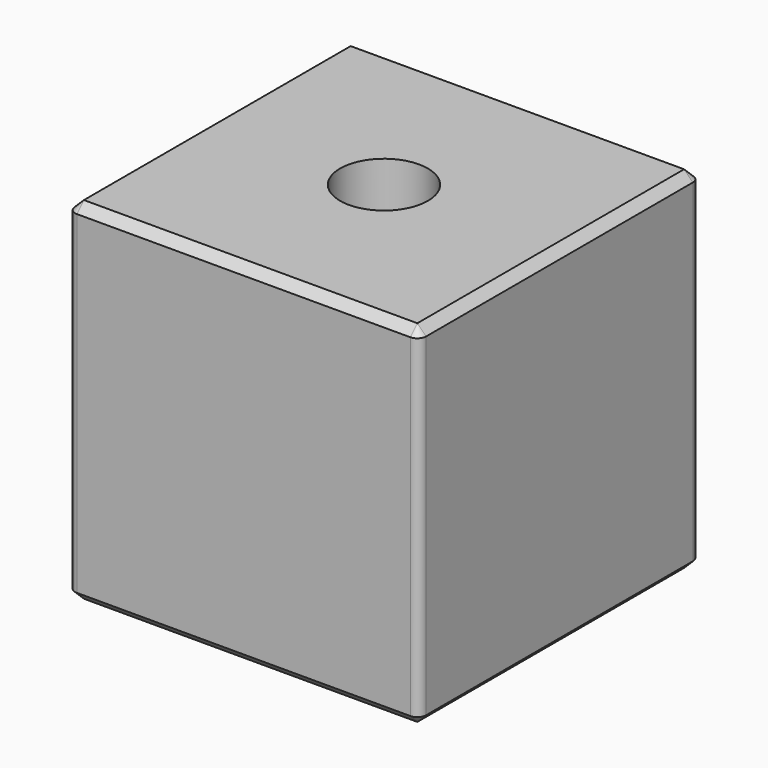
from build123d import *

# Parameters (mm, degrees)
F0_R     = 12.5
F1_DEPTH = 50
F2_SIZE  = 2.49999


# Not quite as in the source:
# - a fillet or chamfer is up to 0.001 mm smaller than in the source, because OpenCascade refuses the exact size


with BuildPart() as f1:
    # F0 (on Top) → F1 (new body, symmetric)
    with BuildSketch(Plane.XY):
        with BuildLine():
            ThreePointArc((-50, -47.5), (-49.267766953, -49.267766953), (-47.5, -50))
            Line((-47.5, -50), (47.5, -50))
            ThreePointArc((47.5, -50), (49.267766953, -49.267766953), (50, -47.5))
            Line((50, -47.5), (50, 47.5))
            ThreePointArc((50, 47.5), (49.267766953, 49.267766953), (47.5, 50))
            Line((47.5, 50), (-47.5, 50))
            ThreePointArc((-47.5, 50), (-49.267766953, 49.267766953), (-50, 47.5))
            Line((-50, 47.5), (-50, -47.5))
        make_face()
        Circle(F0_R, mode=Mode.SUBTRACT)
    extrude(amount=F1_DEPTH, both=True)

    # F2 (size 2.5 in the source; OpenCascade refuses exactly that, so slightly less here)
    f2_edges = [f1.edges().sort_by_distance(p)[0] for p in [
        (50, 0, 50),
        (0, -50, 50),
        (-50, 0, 50),
        (0, 50, 50),
        (50, 0, -50),
        (0, 50, -50),
    ]]
    chamfer(f2_edges, length=F2_SIZE)


solid = f1.part
